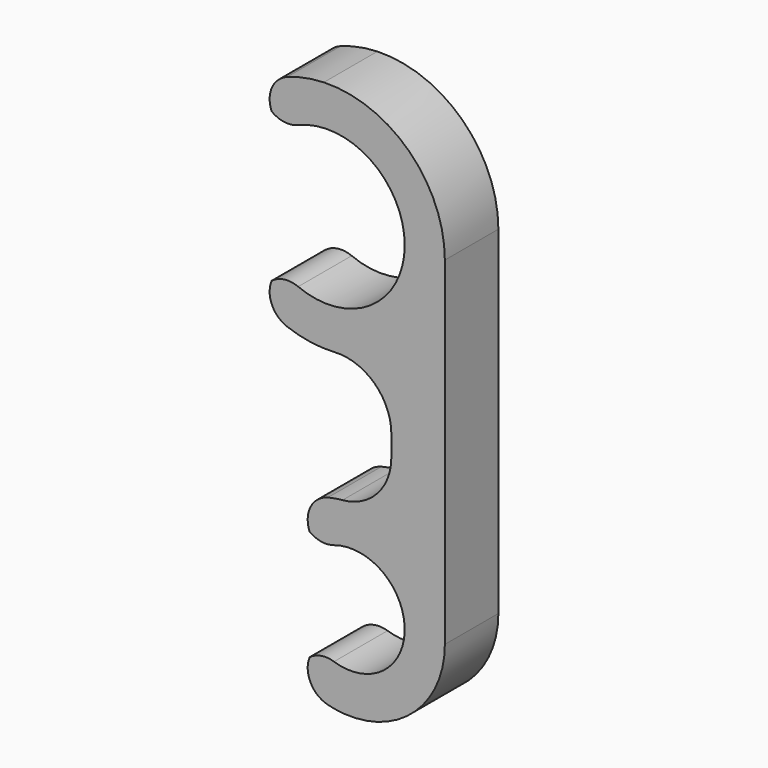
from build123d import *

# Parameters (mm, degrees)
F1_DEPTH    = 5
F2_T1_DEPTH = 18.1085359619
F2_T3_DEPTH = 13.6883237314
F2_T5_DEPTH = 19.2734411819
F2_T7_DEPTH = 13.2933208328


# Not quite as in the source:
# - a fillet or chamfer that OpenCascade refuses, or shapes differently, is made with other operations: its cross-section is extruded or revolved along the edge and cut away or added


with BuildPart() as f1:
    # F0 (on Front) → F1 (new body)
    with BuildSketch(Plane.XZ):
        with BuildLine():
            Line((8.755, -25.285), (8.755, 0))
            ThreePointArc((8.755, 0), (6.0873467679, 6.2923949596), (-0.2899421651, 8.7501976287))
            ThreePointArc((-0.2899421651, 8.7501976287), (-2.9511128894, 8.2426305094), (-5.329706311, 6.9458084942))
            Line((-5.329706311, 6.9458084942), (-3.5034220239, 4.5657484734))
            ThreePointArc((-3.5034220239, 4.5657484734), (5.755, 0), (-3.5034220239, -4.5657484734))
            Line((-3.5034220239, -4.5657484734), (-5.329706311, -6.9458084942))
            ThreePointArc((-5.329706311, -6.9458084942), (-4.2988977903, -7.6268933904), (-3.1824790985, -8.1560929242))
            ThreePointArc((-3.1824790985, -8.1560929242), (-1.3637045363, -8.648140548), (0.5182301058, -8.7396488807))
            ThreePointArc((0.5182301058, -8.7396488807), (3.4984394857, -9.8217007124), (4.755, -12.7326352339))
            Line((4.755, -12.7326352339), (4.755, -14.2977346441))
            ThreePointArc((4.755, -14.2977346441), (3.705175556, -16.9989314509), (1.1067679057, -18.2822370397))
            ThreePointArc((1.1067679057, -18.2822370397), (-0.8255248465, -18.7339906879), (-2.5545928459, -19.7077260178))
            Line((-2.5545928459, -19.7077260178), (-0.7283085589, -22.0877860386))
            ThreePointArc((-0.7283085589, -22.0877860386), (5.755, -25.285), (-0.7283085589, -28.4822139614))
            Line((-0.7283085589, -28.4822139614), (-2.5545928459, -30.8622739822))
            ThreePointArc((-2.5545928459, -30.8622739822), (-0.7476906173, -31.8657827127), (1.2729501298, -32.3004508704))
            ThreePointArc((1.2729501298, -32.3004508704), (6.5334815385, -30.4132945795), (8.755, -25.285))
        make_face()
    extrude(amount=F1_DEPTH)

    # F2: fillet of radius 2 on 8 edges, made by hand

    # F2_s2 → F2_t1 (cut)
    with BuildSketch(Plane.XZ.offset(-6.554267981)):
        with BuildLine():
            ThreePointArc((-3.9278099293, 5.1188215596), (-4.2625544155, 6.8913447905), (-3.0342500285, 8.2123901371))
            ThreePointArc((-3.0342500285, 8.2123901371), (-4.2296570401, 7.6655088757), (-5.329706311, 6.9458084942))
            Line((-5.329706311, 6.9458084942), (-3.9278099293, 5.1188215596))
        make_face()
        with BuildLine():
            ThreePointArc((-3.0342500285, -8.2123901371), (-4.2625544155, -6.8913447905), (-3.9278099293, -5.1188215596))
            Line((-3.9278099293, -5.1188215596), (-5.329706311, -6.9458084942))
            ThreePointArc((-5.329706311, -6.9458084942), (-4.2296570401, -7.6655088757), (-3.0342500285, -8.2123901371))
        make_face()
    extrude(amount=F2_T1_DEPTH, mode=Mode.SUBTRACT)

    # F2_s4 → F2_t3 (cut)
    with BuildSketch(Plane.XZ.offset(-4.3441618657)):
        with BuildLine():
            ThreePointArc((-2.2074106697, 5.3148248452), (-3.4912558515, 5.2297553021), (-4.561245298, 5.9443306041))
            Line((-4.561245298, 5.9443306041), (-3.5034220239, 4.5657484734))
            ThreePointArc((-3.5034220239, 4.5657484734), (-2.8798752345, 4.9826041016), (-2.2074106697, 5.3148248452))
        make_face()
        with BuildLine():
            ThreePointArc((-2.2074106697, -5.3148248452), (-3.4912558515, -5.2297553021), (-4.561245298, -5.9443306041))
            Line((-4.561245298, -5.9443306041), (-3.5034220239, -4.5657484734))
            ThreePointArc((-3.5034220239, -4.5657484734), (-2.8798752345, -4.9826041016), (-2.2074106697, -5.3148248452))
        make_face()
    extrude(amount=F2_T3_DEPTH, mode=Mode.SUBTRACT)

    # F2_s6 → F2_t5 (cut)
    with BuildSketch(Plane.XZ.offset(-7.1367205909)):
        with BuildLine():
            ThreePointArc((0.0158522318, -32.1040698711), (-1.3864892611, -30.8222917209), (-1.084610418, -28.9465555846))
            Line((-1.084610418, -28.9465555846), (-2.5545928459, -30.8622739822))
            ThreePointArc((-2.5545928459, -30.8622739822), (-1.3330660217, -31.6150183417), (0.0158522318, -32.1040698711))
        make_face()
        with BuildLine():
            ThreePointArc((-1.084610418, -21.6234444154), (-1.3864892611, -19.7477082791), (0.0158522318, -18.4659301289))
            ThreePointArc((0.0158522318, -18.4659301289), (-1.3330660217, -18.9549816583), (-2.5545928459, -19.7077260178))
            Line((-2.5545928459, -19.7077260178), (-1.084610418, -21.6234444154))
        make_face()
    extrude(amount=F2_T5_DEPTH, mode=Mode.SUBTRACT)

    # F2_s8 → F2_t7 (cut)
    with BuildSketch(Plane.XZ.offset(-4.1466604164)):
        with BuildLine():
            ThreePointArc((0.4709999062, -21.4550673942), (-0.7422563844, -21.46506549), (-1.7380393272, -20.7718792817))
            Line((-1.7380393272, -20.7718792817), (-0.7283085589, -22.0877860386))
            ThreePointArc((-0.7283085589, -22.0877860386), (-0.1554567483, -21.7206231375), (0.4709999062, -21.4550673942))
        make_face()
        with BuildLine():
            ThreePointArc((-1.7380393272, -29.7981207183), (-0.7422563844, -29.10493451), (0.4709999062, -29.1149326058))
            ThreePointArc((0.4709999062, -29.1149326058), (-0.1554567483, -28.8493768625), (-0.7283085589, -28.4822139614))
            Line((-0.7283085589, -28.4822139614), (-1.7380393272, -29.7981207183))
        make_face()
    extrude(amount=F2_T7_DEPTH, mode=Mode.SUBTRACT)


solid = f1.part
